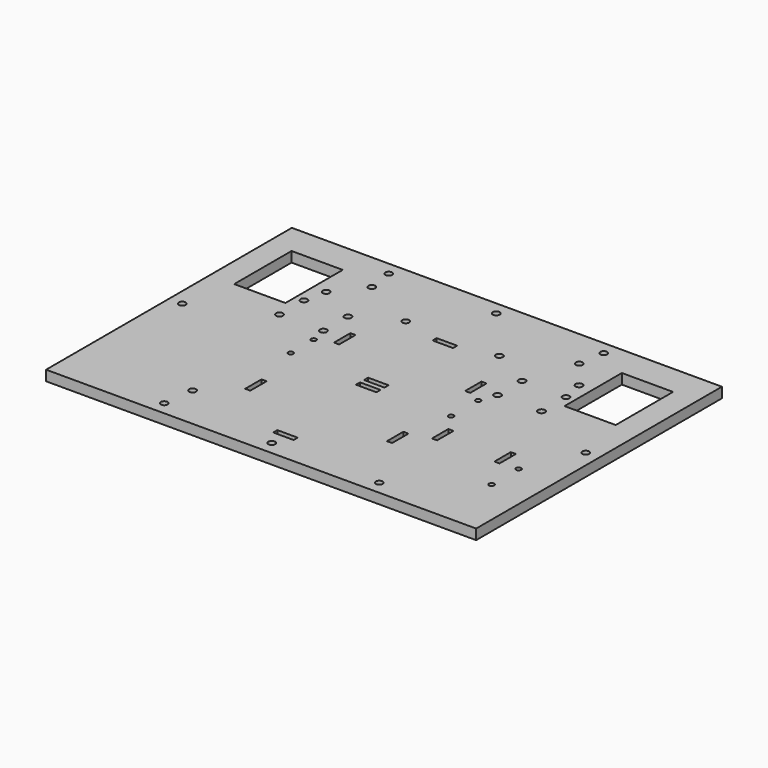
from build123d import *

# Parameters (mm, degrees)
F0_W     = 533.4
F0_H     = 381
F1_DEPTH = 12.7
F5_W     = 25.4
F5_H     = 6.35
F5_W_2   = 6.35
F5_H_2   = 25.4
F5_R     = 3.175
F5_R_2   = 4.28625
F5_R_3   = 4.2926
F5_W_3   = 63.5
F5_H_3   = 88.9
F4_R     = 4.28625
F4_W     = 25.4
F4_H     = 6.35
F4_R_2   = 4.2926
F4_W_2   = 6.35
F4_H_2   = 25.4
F4_W_3   = 63.5
F4_H_3   = 88.9
F6_DEPTH = 12.701


# Not quite as in the source:
# - a feature of the source that left no trace in its solid (it failed there, or was rolled back) is left out


with BuildPart() as f1:
    # F0 (on Top) → F1 (new body)
    with BuildSketch(Plane.XY):
        Rectangle(F0_W, F0_H)
    extrude(amount=F1_DEPTH)

    # F5 (on face) + F4 (on face) → F6 (cut, through all)
    with BuildSketch(Plane.XY.offset(12.7)):
        with Locations((0, -24.4856)):
            Rectangle(F5_W, F5_H)
        with Locations((87.9475, -88.6206)):
            Rectangle(F5_W_2, F5_H_2)
        with Locations((0, -152.7556)):
            Rectangle(F5_W, F5_H)
        with Locations((-87.9475, -88.6206)):
            Rectangle(F5_W_2, F5_H_2)
        with Locations((-103.575, 20.447)):
            Circle(F5_R)
        with Locations((-103.575, -15.113)):
            Circle(F5_R)
        with Locations((220.6625, -67.183)):
            Circle(F5_R)
        with Locations((220.6625, -109.093)):
            Circle(F5_R)
        with Locations((100.4, 20.447)):
            Circle(F5_R)
        with Locations((100.4, -21.463)):
            Circle(F5_R)
        with Locations((118.4275, -57.023)):
            Rectangle(F5_W_2, F5_H_2)
        with Locations((195.8975, -57.023)):
            Rectangle(F5_W_2, F5_H_2)
        with Locations((-128.6256, -135.89)):
            Circle(F5_R_2)
        with Locations((0, -11.938)):
            Rectangle(F5_W, F5_H)
        with Locations((-162.4810314, 41.0845)):
            Circle(F5_R_3)
        with Locations((-162.4810314, 79.0575)):
            Circle(F5_R_3)
        with Locations((-108.0289686, 41.0845)):
            Circle(F5_R_3)
        with Locations((-81.28, 40.767)):
            Rectangle(F5_W_2, F5_H_2)
        with Locations((-108.0289686, 79.0575)):
            Circle(F5_R_3)
        with Locations((-204.8256, 107.95)):
            Rectangle(F5_W_3, F5_H_3)
        with Locations((-156.810075, 106.3625)):
            Circle(F5_R_3)
        with Locations((-128.6256, 141.9225)):
            Circle(F5_R_2)
        with Locations((-58.0445372, 106.3625)):
            Circle(F5_R_2)
        with Locations((81.28, 40.767)):
            Rectangle(F5_W_2, F5_H_2)
        with Locations((108.0289686, 41.0845)):
            Circle(F5_R_3)
        with Locations((0, 94.2975)):
            Rectangle(F5_W, F5_H)
        with Locations((108.0289686, 79.0575)):
            Circle(F5_R_3)
        with Locations((162.4810314, 41.0845)):
            Circle(F5_R_3)
        with Locations((162.4810314, 79.0575)):
            Circle(F5_R_3)
        with Locations((58.0445372, 106.3625)):
            Circle(F5_R_2)
        with Locations((128.6256, 141.9225)):
            Circle(F5_R_2)
        with Locations((156.810075, 106.3625)):
            Circle(F5_R_3)
        with Locations((204.8256, 107.95)):
            Rectangle(F5_W_3, F5_H_3)
    with BuildSketch(Plane.XY.offset(12.7)):
        with Locations((-133.35, 173.99)):
            Circle(F4_R)
        with Locations((0, 173.99)):
            Circle(F4_R)
        with Locations((133.35, 173.99)):
            Circle(F4_R)
        with Locations((250.19, 0)):
            Circle(F4_R)
        with Locations((-250.19, 0)):
            Circle(F4_R)
        with Locations((0, -173.99)):
            Circle(F4_R)
        with Locations((133.35, -173.99)):
            Circle(F4_R)
        with Locations((-133.35, -173.99)):
            Circle(F4_R)
        with Locations((-128.6256, -135.89)):
            Circle(F4_R)
        with Locations((0, -11.938)):
            Rectangle(F4_W, F4_H)
        with Locations((-162.4810314, 41.0845)):
            Circle(F4_R_2)
        with Locations((-162.4810314, 79.0575)):
            Circle(F4_R_2)
        with Locations((-108.0289686, 41.0845)):
            Circle(F4_R_2)
        with Locations((-81.28, 40.767)):
            Rectangle(F4_W_2, F4_H_2)
        with Locations((-108.0289686, 79.0575)):
            Circle(F4_R_2)
        with Locations((-204.8256, 107.95)):
            Rectangle(F4_W_3, F4_H_3)
        with Locations((-156.810075, 106.3625)):
            Circle(F4_R_2)
        with Locations((-128.6256, 141.9225)):
            Circle(F4_R)
        with Locations((-58.0445372, 106.3625)):
            Circle(F4_R)
        with Locations((81.28, 40.767)):
            Rectangle(F4_W_2, F4_H_2)
        with Locations((108.0289686, 41.0845)):
            Circle(F4_R_2)
        with Locations((0, 94.2975)):
            Rectangle(F4_W, F4_H)
        with Locations((108.0289686, 79.0575)):
            Circle(F4_R_2)
        with Locations((162.4810314, 41.0845)):
            Circle(F4_R_2)
        with Locations((162.4810314, 79.0575)):
            Circle(F4_R_2)
        with Locations((58.0445372, 106.3625)):
            Circle(F4_R)
        with Locations((128.6256, 141.9225)):
            Circle(F4_R)
        with Locations((156.810075, 106.3625)):
            Circle(F4_R_2)
        with Locations((204.8256, 107.95)):
            Rectangle(F4_W_3, F4_H_3)
    extrude(amount=-F6_DEPTH, mode=Mode.SUBTRACT)


solid = f1.part
